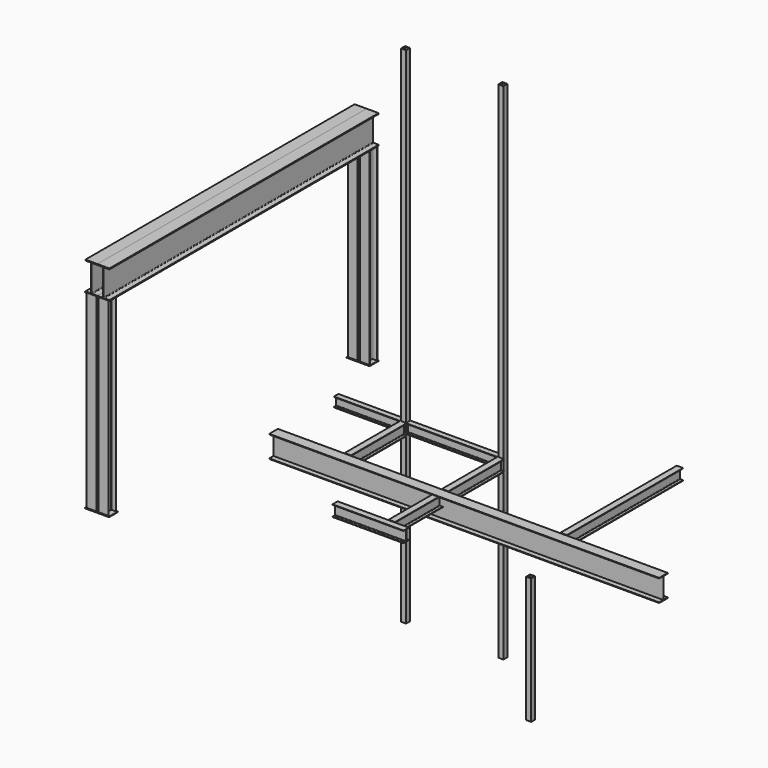
from build123d import *

# Parameters (mm, degrees)
F0_W           = 80
F0_H           = 80
F0_W_2         = 64
F0_H_2         = 64
F1_DEPTH       = 8000
F2_DEPTH       = 2000
F10_DEPTH      = 2000
F10_DEPTH_BACK = 4180
F13_DEPTH      = 2287
F13_DEPTH_BACK = 100
F15_DEPTH      = 4570.9259889374
F17_DEPTH      = 1187
F19_DEPTH      = 2692.601
F22_DEPTH      = 1462
F24_DEPTH      = 1060
F27_DEPTH      = 1126
F30_DEPTH      = 3000
F34_DEPTH      = 5332.6
F35_W          = 382.9
F35_H          = 177.6
F36_DEPTH      = 10
F35_W_2        = 362.9
F41_DEPTH      = 995.9
F43_DEPTH      = 2969.051


with BuildPart() as f1:
    # F0 (on Top) → F1 (new body)
    with BuildSketch(Plane.XY):
        with Locations((-1000, 0)):
            Rectangle(F0_W, F0_H)
        with Locations((-1000, 0)):
            Rectangle(F0_W_2, F0_H_2, mode=Mode.SUBTRACT)
    extrude(amount=F1_DEPTH)


with BuildPart() as f1b:
    # F0 (on Top) → F1, piece 2 (new body)
    with BuildSketch(Plane.XY):
        with Locations((542, 0)):
            Rectangle(F0_W, F0_H)
        with Locations((542, 0)):
            Rectangle(F0_W_2, F0_H_2, mode=Mode.SUBTRACT)
    extrude(amount=F1_DEPTH)


with BuildPart() as f2:
    # F0 (on Top) → F2 (new body)
    with BuildSketch(Plane.XY):
        with Locations((1855, -1090)):
            Rectangle(F0_W, F0_H)
        with Locations((1855, -1090)):
            Rectangle(F0_W_2, F0_H_2, mode=Mode.SUBTRACT)
    extrude(amount=F2_DEPTH)


with BuildPart() as f10:
    # F9 (on offset) → F10 (new body, two sides)
    with BuildSketch(Plane.YZ.offset(2080)) as f10_sk:
        Polygon((-1154.4499414902, 2800), (-1325.5499414902, 2800), (-1325.5499414902, 2790.3), (-1243.4999414902, 2790.3), (-1243.4999414902, 2458.3), (-1325.5499414902, 2458.3), (-1325.5499414902, 2448.6), (-1154.4499414902, 2448.6), (-1154.4499414902, 2458.3), (-1236.4999414902, 2458.3), (-1236.4999414902, 2790.3), (-1154.4499414902, 2790.3), align=None)
    extrude(amount=F10_DEPTH)
    extrude(f10_sk.sketch, amount=-F10_DEPTH_BACK)


with BuildPart() as f13:
    # F12 (on offset) → F13 (new body, two sides)
    with BuildSketch(Plane.XZ.offset(-1060)) as f13_sk:
        with BuildLine():
            Line((2470.9249889374, 2792.1), (2470.9249889374, 2800))
            Line((2470.9249889374, 2800), (2369.7249889374, 2800))
            Line((2369.7249889374, 2800), (2369.7249889374, 2792.1))
            Line((2369.7249889374, 2792.1), (2410.3249889374, 2792.1))
            ThreePointArc((2410.3249889374, 2792.1), (2415.6990004744, 2789.874011537), (2417.9249889374, 2784.5))
            Line((2417.9249889374, 2784.5), (2417.9249889374, 2637.7))
            ThreePointArc((2417.9249889374, 2637.7), (2415.6990004744, 2632.325988463), (2410.3249889374, 2630.1))
            Line((2410.3249889374, 2630.1), (2369.7249889374, 2630.1))
            Line((2369.7249889374, 2630.1), (2369.7249889374, 2622.2))
            Line((2369.7249889374, 2622.2), (2470.9249889374, 2622.2))
            Line((2470.9249889374, 2622.2), (2470.9249889374, 2630.1))
            Line((2470.9249889374, 2630.1), (2430.3249889374, 2630.1))
            ThreePointArc((2430.3249889374, 2630.1), (2424.9509774004, 2632.325988463), (2422.7249889374, 2637.7))
            Line((2422.7249889374, 2637.7), (2422.7249889374, 2784.5))
            ThreePointArc((2422.7249889374, 2784.5), (2424.9509774004, 2789.874011537), (2430.3249889374, 2792.1))
            Line((2430.3249889374, 2792.1), (2470.9249889374, 2792.1))
        make_face()
    extrude(amount=F13_DEPTH)
    extrude(f13_sk.sketch, amount=-F13_DEPTH_BACK)

    # F14 (on face) → F15 (cut, through all)
    with BuildSketch(Plane.YZ.offset(2470.9249889374)):
        with BuildLine():
            Line((-1227, 2800), (-1227, 2780.3))
            Line((-1227, 2780.3), (-1154.4499414902, 2780.3))
            ThreePointArc((-1154.4499414902, 2780.3), (-1147.3788736783, 2783.2289321881), (-1144.4499414902, 2790.3))
            Line((-1144.4499414902, 2790.3), (-1144.4499414902, 2800))
            Line((-1144.4499414902, 2800), (-1227, 2800))
        make_face()
    extrude(amount=-F15_DEPTH, mode=Mode.SUBTRACT)


with BuildPart() as f17:
    # F16 (on face) → F17 (new body)
    with BuildSketch(Plane.XZ.offset(40)):
        with BuildLine():
            Line((592.6, 2792.1), (592.6, 2800))
            Line((592.6, 2800), (491.4, 2800))
            Line((491.4, 2800), (491.4, 2792.1))
            Line((491.4, 2792.1), (530.8, 2792.1))
            ThreePointArc((530.8, 2792.1), (536.174011537, 2789.874011537), (538.4, 2784.5))
            Line((538.4, 2784.5), (538.4, 2637.7))
            ThreePointArc((538.4, 2637.7), (536.174011537, 2632.325988463), (530.8, 2630.1))
            Line((530.8, 2630.1), (491.4, 2630.1))
            Line((491.4, 2630.1), (491.4, 2622.2))
            Line((491.4, 2622.2), (592.6, 2622.2))
            Line((592.6, 2622.2), (592.6, 2630.1))
            Line((592.6, 2630.1), (553.2, 2630.1))
            ThreePointArc((553.2, 2630.1), (547.825988463, 2632.325988463), (545.6, 2637.7))
            Line((545.6, 2637.7), (545.6, 2784.5))
            ThreePointArc((545.6, 2784.5), (547.825988463, 2789.874011537), (553.2, 2792.1))
            Line((553.2, 2792.1), (592.6, 2792.1))
        make_face()
    extrude(amount=F17_DEPTH)

    # F18 (on face) → F19 (cut, through all)
    with BuildSketch(Plane.YZ.offset(592.6)):
        with BuildLine():
            Line((-1144.45, 2800), (-1227, 2800))
            Line((-1227, 2800), (-1227, 2780.3))
            Line((-1227, 2780.3), (-1154.45, 2780.3))
            ThreePointArc((-1154.45, 2780.3), (-1147.3789321881, 2783.2289321881), (-1144.45, 2790.3))
            Line((-1144.45, 2790.3), (-1144.45, 2800))
        make_face()
    extrude(amount=-F19_DEPTH, mode=Mode.SUBTRACT)


with BuildPart() as f20_1:
    # F20: copy of F17
    add(f17.part.moved(Location((-1542, 0, 0))))


with BuildPart() as f22:
    # F21 (on face) → F22 (new body)
    with BuildSketch(Plane.YZ.offset(-960)):
        with BuildLine():
            Line((44.35, 2800), (-44.35, 2800))
            Line((-44.35, 2800), (-44.35, 2792.3))
            Line((-44.35, 2792.3), (-9.85, 2792.3))
            ThreePointArc((-9.85, 2792.3), (-4.475988463, 2790.074011537), (-2.25, 2784.7))
            Line((-2.25, 2784.7), (-2.25, 2662.9))
            ThreePointArc((-2.25, 2662.9), (-4.475988463, 2657.525988463), (-9.85, 2655.3))
            Line((-9.85, 2655.3), (-44.35, 2655.3))
            Line((-44.35, 2655.3), (-44.35, 2647.6))
            Line((-44.35, 2647.6), (44.35, 2647.6))
            Line((44.35, 2647.6), (44.35, 2655.3))
            Line((44.35, 2655.3), (9.85, 2655.3))
            ThreePointArc((9.85, 2655.3), (4.475988463, 2657.525988463), (2.25, 2662.9))
            Line((2.25, 2662.9), (2.25, 2784.7))
            ThreePointArc((2.25, 2784.7), (4.475988463, 2790.074011537), (9.85, 2792.3))
            Line((9.85, 2792.3), (44.35, 2792.3))
            Line((44.35, 2792.3), (44.35, 2800))
        make_face()
    extrude(amount=F22_DEPTH)


with BuildPart() as f24:
    # F23 (on face) → F24 (new body)
    with BuildSketch(Plane(origin=(-1040, 0, 0), x_dir=(0, -1, 0), z_dir=(-1, 0, 0))):
        with BuildLine():
            Line((-40, 2800), (-44.35, 2800))
            Line((-44.35, 2800), (-44.35, 2792.3))
            Line((-44.35, 2792.3), (-9.85, 2792.3))
            ThreePointArc((-9.85, 2792.3), (-4.475988463, 2790.074011537), (-2.25, 2784.7))
            Line((-2.25, 2784.7), (-2.25, 2662.9))
            ThreePointArc((-2.25, 2662.9), (-4.475988463, 2657.525988463), (-9.85, 2655.3))
            Line((-9.85, 2655.3), (-44.35, 2655.3))
            Line((-44.35, 2655.3), (-44.35, 2647.6))
            Line((-44.35, 2647.6), (0, 2647.6))
            Line((0, 2647.6), (0, 2800))
            Line((0, 2800), (-40, 2800))
        make_face()
        with BuildLine():
            Line((40, 2800), (0, 2800))
            Line((0, 2800), (0, 2647.6))
            Line((0, 2647.6), (44.35, 2647.6))
            Line((44.35, 2647.6), (44.35, 2655.3))
            Line((44.35, 2655.3), (9.85, 2655.3))
            ThreePointArc((9.85, 2655.3), (4.475988463, 2657.525988463), (2.25, 2662.9))
            Line((2.25, 2662.9), (2.25, 2784.7))
            ThreePointArc((2.25, 2784.7), (4.475988463, 2790.074011537), (9.85, 2792.3))
            Line((9.85, 2792.3), (44.35, 2792.3))
            Line((44.35, 2792.3), (44.35, 2800))
            Line((44.35, 2800), (40, 2800))
        make_face()
    extrude(amount=F24_DEPTH)


with BuildPart() as f27:
    # F26 (on offset) → F27 (new body)
    with BuildSketch(Plane.YZ.offset(817)):
        with BuildLine():
            Line((-2209.3999414902, 2792.1), (-2209.3999414902, 2800))
            Line((-2209.3999414902, 2800), (-2310.5999414902, 2800))
            Line((-2310.5999414902, 2800), (-2310.5999414902, 2792.1))
            Line((-2310.5999414902, 2792.1), (-2269.9999414902, 2792.1))
            ThreePointArc((-2269.9999414902, 2792.1), (-2266.2355274872, 2789.3341196033), (-2264.7999414902, 2784.8888974491))
            Line((-2264.7999414902, 2784.8888974491), (-2264.7999414902, 2637.7))
            ThreePointArc((-2264.7999414902, 2637.7), (-2267.0259299532, 2632.325988463), (-2272.3999414902, 2630.1))
            Line((-2272.3999414902, 2630.1), (-2310.5999414902, 2630.1))
            Line((-2310.5999414902, 2630.1), (-2310.5999414902, 2622.2))
            Line((-2310.5999414902, 2622.2), (-2209.3999414902, 2622.2))
            Line((-2209.3999414902, 2622.2), (-2209.3999414902, 2630.1))
            Line((-2209.3999414902, 2630.1), (-2249.9999414902, 2630.1))
            ThreePointArc((-2249.9999414902, 2630.1), (-2255.3739530272, 2632.325988463), (-2257.5999414902, 2637.7))
            Line((-2257.5999414902, 2637.7), (-2257.5999414902, 2784.5))
            ThreePointArc((-2257.5999414902, 2784.5), (-2255.3739530272, 2789.874011537), (-2249.9999414902, 2792.1))
            Line((-2249.9999414902, 2792.1), (-2209.3999414902, 2792.1))
        make_face()
    extrude(amount=-F27_DEPTH)


with BuildPart() as f30:
    # F29 (on offset) → F30 (new body)
    with BuildSketch(Plane.XY.offset(3025)):
        with BuildLine():
            Line((-2280, 631.0000585098), (-2277.1, 631.0000585098))
            Line((-2277.1, 631.0000585098), (-2277.1, 695.4000585098))
            ThreePointArc((-2277.1, 695.4000585098), (-2274.874011537, 700.7740700468), (-2269.5, 703.0000585098))
            Line((-2269.5, 703.0000585098), (-2203.55, 703.0000585098))
            Line((-2203.55, 703.0000585098), (-2203.55, 709.8000585098))
            Line((-2203.55, 709.8000585098), (-2280, 709.8000585098))
            Line((-2280, 709.8000585098), (-2280, 631.0000585098))
        make_face()
        with BuildLine():
            Line((-2282.9, 631.0000585098), (-2280, 631.0000585098))
            Line((-2280, 631.0000585098), (-2280, 709.8000585098))
            Line((-2280, 709.8000585098), (-2356.45, 709.8000585098))
            Line((-2356.45, 709.8000585098), (-2356.45, 703.0000585098))
            Line((-2356.45, 703.0000585098), (-2290.5, 703.0000585098))
            ThreePointArc((-2290.5, 703.0000585098), (-2285.125988463, 700.7740700468), (-2282.9, 695.4000585098))
            Line((-2282.9, 695.4000585098), (-2282.9, 631.0000585098))
        make_face()
        with BuildLine():
            Line((-2280, 552.2000585098), (-2280, 631.0000585098))
            Line((-2280, 631.0000585098), (-2282.9, 631.0000585098))
            Line((-2282.9, 631.0000585098), (-2282.9, 566.6000585098))
            ThreePointArc((-2282.9, 566.6000585098), (-2285.125988463, 561.2260469728), (-2290.5, 559.0000585098))
            Line((-2290.5, 559.0000585098), (-2356.45, 559.0000585098))
            Line((-2356.45, 559.0000585098), (-2356.45, 552.2000585098))
            Line((-2356.45, 552.2000585098), (-2280, 552.2000585098))
        make_face()
        with BuildLine():
            Line((-2277.1, 566.6000585098), (-2277.1, 631.0000585098))
            Line((-2277.1, 631.0000585098), (-2280, 631.0000585098))
            Line((-2280, 631.0000585098), (-2280, 552.2000585098))
            Line((-2280, 552.2000585098), (-2203.55, 552.2000585098))
            Line((-2203.55, 552.2000585098), (-2203.55, 559.0000585098))
            Line((-2203.55, 559.0000585098), (-2269.5, 559.0000585098))
            ThreePointArc((-2269.5, 559.0000585098), (-2274.874011537, 561.2260469728), (-2277.1, 566.6000585098))
        make_face()
    extrude(amount=F30_DEPTH)


with BuildPart() as f31_1:
    # F31: copy of F30
    add(f30.part.moved(Location((190, 0, 0))))


with BuildPart() as f32_1:
    # F32: copy of F30
    add(f30.part.moved(Location((0, -5175, 0))))


with BuildPart() as f32_2:
    # F32: copy of F31_1
    add(f31_1.part.moved(Location((0, -5175, 0))))


with BuildPart() as f34:
    # F33 (on face) → F34 (new body)
    with BuildSketch(Plane.XZ.offset(4622.7999414902)):
        with BuildLine():
            Line((-1995.828, 6482), (-2185.828, 6482))
            Line((-2185.828, 6482), (-2185.828, 6467.5))
            Line((-2185.828, 6467.5), (-2105.528, 6467.5))
            ThreePointArc((-2105.528, 6467.5), (-2098.3155108319, 6464.5124891681), (-2095.328, 6457.3))
            Line((-2095.328, 6457.3), (-2095.328, 6049.7))
            ThreePointArc((-2095.328, 6049.7), (-2098.3155108319, 6042.4875108319), (-2105.528, 6039.5))
            Line((-2105.528, 6039.5), (-2185.828, 6039.5))
            Line((-2185.828, 6039.5), (-2185.828, 6025))
            Line((-2185.828, 6025), (-1995.828, 6025))
            Line((-1995.828, 6025), (-1995.828, 6039.5))
            Line((-1995.828, 6039.5), (-2076.128, 6039.5))
            ThreePointArc((-2076.128, 6039.5), (-2083.3404891681, 6042.4875108319), (-2086.328, 6049.7))
            Line((-2086.328, 6049.7), (-2086.328, 6457.3))
            ThreePointArc((-2086.328, 6457.3), (-2083.3404891681, 6464.5124891681), (-2076.128, 6467.5))
            Line((-2076.128, 6467.5), (-1995.828, 6467.5))
            Line((-1995.828, 6467.5), (-1995.828, 6482))
        make_face()
    extrude(amount=-F34_DEPTH)


with BuildPart() as f36:
    # F35 (on face) → F36 (new body)
    with BuildSketch(Plane.XY.offset(6025)):
        with Locations((-2185, -4543.9999414902)):
            Rectangle(F35_W, F35_H)
    extrude(amount=F36_DEPTH)


with BuildPart() as f36b:
    # F35 (on face) → F36, piece 2 (new body)
    with BuildSketch(Plane.XY.offset(6025)):
        with Locations((-2185, 631.0000585098)):
            Rectangle(F35_W_2, F35_H)
    extrude(amount=F36_DEPTH)


with BuildPart() as f37_1:
    # F37: copy of F34
    add(f34.part.moved(Location((-190, 0, 0))))


with BuildPart() as f38_1:
    # F38: copy of F36
    add(f36.part.moved(Location((0, 0, -3010))))


with BuildPart() as f38_2:
    # F38: copy of F36b
    add(f36b.part.moved(Location((0, 0, -3010))))


with BuildPart() as f41:
    # F40 (on offset) → F41 (new body)
    with BuildSketch(Plane.XZ.offset(1253.4999414902)):
        with BuildLine():
            Line((592.6, 2792.1), (592.6, 2800))
            Line((592.6, 2800), (491.4, 2800))
            Line((491.4, 2800), (491.4, 2792.1))
            Line((491.4, 2792.1), (532, 2792.1))
            ThreePointArc((532, 2792.1), (537.374011537, 2789.874011537), (539.6, 2784.5))
            Line((539.6, 2784.5), (539.6, 2637.7))
            ThreePointArc((539.6, 2637.7), (537.374011537, 2632.325988463), (532, 2630.1))
            Line((532, 2630.1), (491.4, 2630.1))
            Line((491.4, 2630.1), (491.4, 2622.2))
            Line((491.4, 2622.2), (592.6, 2622.2))
            Line((592.6, 2622.2), (592.6, 2630.1))
            Line((592.6, 2630.1), (552, 2630.1))
            ThreePointArc((552, 2630.1), (546.625988463, 2632.325988463), (544.4, 2637.7))
            Line((544.4, 2637.7), (544.4, 2784.5))
            ThreePointArc((544.4, 2784.5), (546.625988463, 2789.874011537), (552, 2792.1))
            Line((552, 2792.1), (592.6, 2792.1))
        make_face()
    extrude(amount=F41_DEPTH)

    # F42 (on face) → F43 (cut, through all)
    with BuildSketch(Plane.YZ.offset(592.6)):
        with BuildLine():
            Line((-2199.3999414902, 2800), (-2249.3999414902, 2800))
            Line((-2249.3999414902, 2800), (-2249.3999414902, 2782.1))
            Line((-2249.3999414902, 2782.1), (-2209.3999414902, 2782.1))
            ThreePointArc((-2209.3999414902, 2782.1), (-2202.3288736783, 2785.0289321881), (-2199.3999414902, 2792.1))
            Line((-2199.3999414902, 2792.1), (-2199.3999414902, 2800))
        make_face()
        with BuildLine():
            Line((-2209.3999414902, 2640.1), (-2249.3999414902, 2640.1))
            Line((-2249.3999414902, 2640.1), (-2249.3999414902, 1621.6330505371))
            Line((-2249.3999414902, 1621.6330505371), (-2199.3999414902, 1621.6330505371))
            Line((-2199.3999414902, 1621.6330505371), (-2199.3999414902, 2630.1))
            ThreePointArc((-2199.3999414902, 2630.1), (-2202.3288736783, 2637.1710678119), (-2209.3999414902, 2640.1))
        make_face()
        with BuildLine():
            Line((-1252.1662621002, 2800), (-1335.5499414902, 2800))
            Line((-1335.5499414902, 2800), (-1335.5499414902, 2790.3))
            ThreePointArc((-1335.5499414902, 2790.3), (-1332.621009302, 2783.2289321881), (-1325.5499414902, 2780.3))
            Line((-1325.5499414902, 2780.3), (-1252.1662621002, 2780.3))
            Line((-1252.1662621002, 2780.3), (-1252.1662621002, 2800))
        make_face()
    extrude(amount=-F43_DEPTH, mode=Mode.SUBTRACT)


solid = Compound([f1.part, f1b.part, f2.part, f10.part, f13.part, f17.part, f20_1.part, f22.part, f24.part, f27.part, f30.part, f31_1.part, f32_1.part, f32_2.part, f34.part, f36.part, f36b.part, f37_1.part, f38_1.part, f38_2.part, f41.part])
